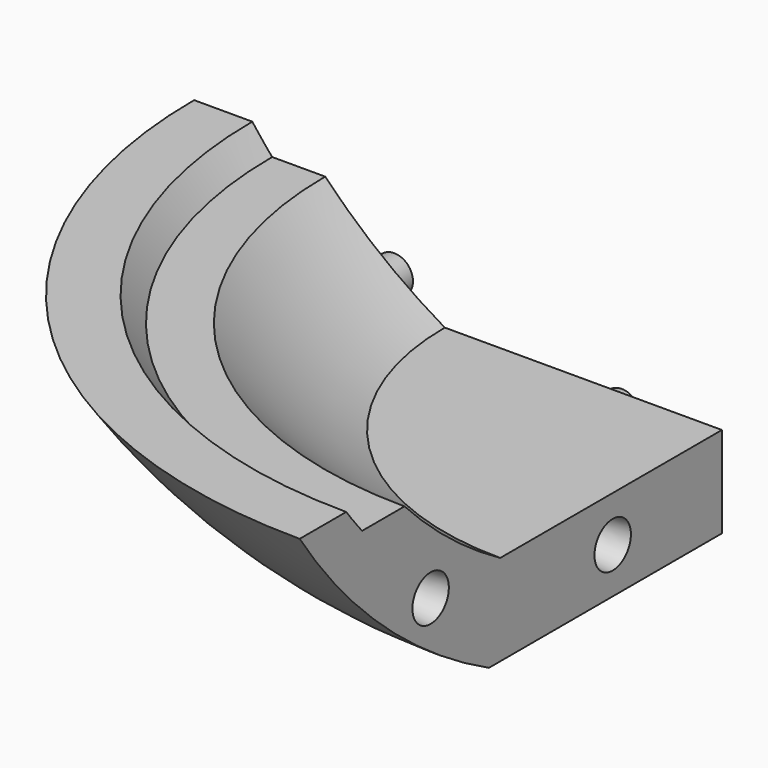
from build123d import *

# Parameters (mm, degrees)
F1_ANGLE = 90
F3_R     = 6.35
F4_DEPTH = 12.7
F4_TAPER = 5
F5_R     = 6.35
F6_DEPTH = 12.7
F6_TAPER = 5


# Not quite as in the source:
# - a feature of the source that left no trace in its solid (it failed there, or was rolled back) is left out


with BuildPart() as f1:
    # F0 (on Front) → F1 (revolve)
    with BuildSketch(Plane.XZ):
        with BuildLine():
            Line((-81.28, -158.1341253493), (0, -158.1341253493))
            Line((0, -158.1341253493), (0, -132.7341253493))
            Line((0, -132.7341253493), (-77.331499878, -132.7341253493))
            ThreePointArc((-77.331499878, -132.7341253493), (-94.9330399433, -120.7734525165), (-110.7127485092, -106.4950525761))
            Line((-110.7127485092, -106.4950525761), (-125.4562139511, -106.4950525761))
            Line((-125.4562139511, -106.4950525761), (-125.5056119373, -106.4950525761))
            ThreePointArc((-125.5056119373, -106.4950525761), (-128.3196475153, -103.0869677141), (-131.041165147, -99.6045575657))
            Line((-131.041165147, -99.6045575657), (-147.2812687077, -99.6045575657))
            ThreePointArc((-147.2812687077, -99.6045575657), (-117.9681777623, -133.0276250839), (-81.28, -158.1341253493))
        make_face()
    revolve(axis=Axis((0, 0, -145.4341253493), (0, 0, 1)), revolution_arc=F1_ANGLE)

    # F3 (on face) → F4 (join)
    with BuildSketch(Plane.XZ):
        with Locations((-101.6, -132.7341253493)):
            Circle(F3_R)
        with Locations((-38.1, -145.4341253493)):
            Circle(F3_R)
    extrude(amount=-F4_DEPTH, taper=F4_TAPER)

    # F5 (on face) → F6 (cut)
    with BuildSketch(Plane.YZ):
        with Locations((-101.6, -132.7341253493)):
            Circle(F5_R)
        with Locations((-38.1, -145.4341253493)):
            Circle(F5_R)
    extrude(amount=-F6_DEPTH, taper=F6_TAPER, mode=Mode.SUBTRACT)


solid = f1.part
